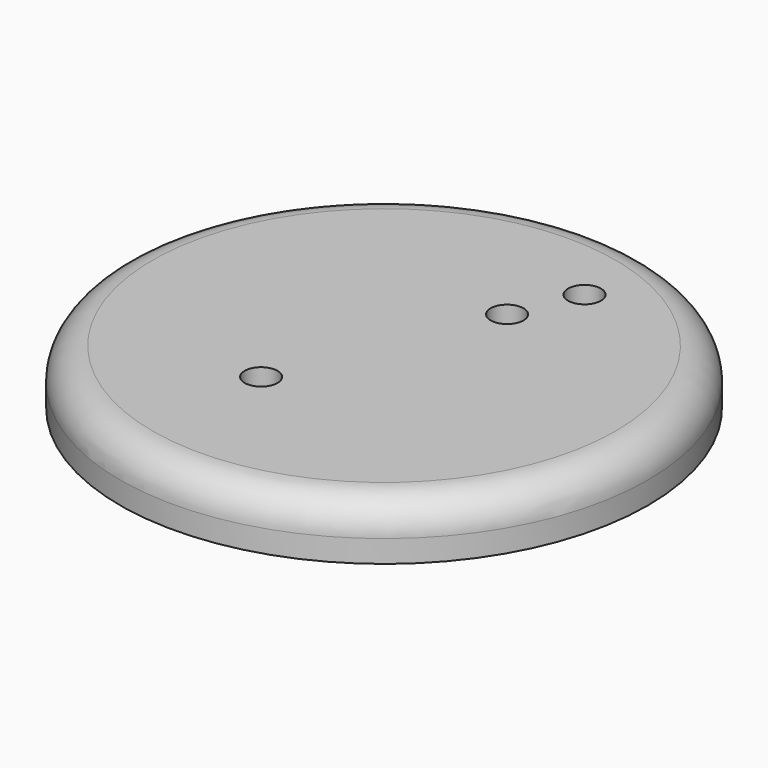
from build123d import *

# Parameters (mm, degrees)
F0_R           = 65
F1_DEPTH       = 15
F2_R           = 8
F3_R           = 60
F3_R_2         = 54
F4_DEPTH       = 3
F5_R           = 8
F6_DEPTH       = 10
F9_R           = 1.5
F10_DEPTH      = 55.0000001083
F10_DEPTH_BACK = 55.0000001083
F11_R          = 1.5
F12_DEPTH      = 55.0000001
F12_DEPTH_BACK = 55.0000000958
F13_R          = 1.5
F14_DEPTH      = 55.0000001083
F14_DEPTH_BACK = 55.0000001083
F15_R          = 1.5
F16_DEPTH      = 55.0000001083
F16_DEPTH_BACK = 55.0000001083
F17_R          = 8
F17_R_2        = 5.75
F18_DEPTH      = 4
F19_R          = 1.75
F20_DEPTH      = 10
F21_R          = 4.05
F22_DEPTH      = 15.001
F23_R          = 8.1
F24_DEPTH      = 7.1
F25_R          = 3.5
F26_DEPTH      = 8
F27_R          = 65
F27_R_2        = 60
F28_DEPTH      = 1.5
F29_SIZE       = 1.49999


# Not quite as in the source:
# - a fillet or chamfer is up to 0.001 mm smaller than in the source, because OpenCascade refuses the exact size


with BuildPart() as f1:
    # F0 (on Top) → F1 (new body)
    with BuildSketch(Plane.XY):
        Circle(F0_R)
    extrude(amount=F1_DEPTH)

    # F2
    f2_edges = [f1.edges().sort_by_distance(p)[0] for p in [
        (-65, 0, 15),
    ]]
    fillet(f2_edges, radius=F2_R)

    # F3 (on face) → F4 (cut)
    with BuildSketch(Plane(origin=(0, 0, 0), x_dir=(1, 0, 0), z_dir=(0, 0, -1))):
        Circle(F3_R)
        Circle(F3_R_2, mode=Mode.SUBTRACT)
    extrude(amount=-F4_DEPTH, mode=Mode.SUBTRACT)

    # F5 (on face) → F6 (cut)
    with BuildSketch(Plane(origin=(0, 0, 0), x_dir=(1, 0, 0), z_dir=(0, 0, -1))):
        Circle(F5_R)
    extrude(amount=-F6_DEPTH, mode=Mode.SUBTRACT)

    # F9 (on Front) → F10 (cut, two sides)
    with BuildSketch(Plane.XZ) as f10_sk:
        Circle(F9_R)
    extrude(amount=-F10_DEPTH, mode=Mode.SUBTRACT)
    extrude(f10_sk.sketch, amount=F10_DEPTH_BACK, mode=Mode.SUBTRACT)

    # F11 (on Right) → F12 (cut, two sides)
    with BuildSketch(Plane.YZ) as f12_sk:
        Circle(F11_R)
    extrude(amount=F12_DEPTH, mode=Mode.SUBTRACT)
    extrude(f12_sk.sketch, amount=-F12_DEPTH_BACK, mode=Mode.SUBTRACT)

    # F13 (on face) → F14 (cut, two sides)
    with BuildSketch(Plane(origin=(0, 0, 0), x_dir=(0.7071067812, -0.7071067812, 0), z_dir=(-0.7071067812, -0.7071067812, 0))) as f14_sk:
        Circle(F13_R)
    extrude(amount=-F14_DEPTH, mode=Mode.SUBTRACT)
    extrude(f14_sk.sketch, amount=F14_DEPTH_BACK, mode=Mode.SUBTRACT)

    # F15 (on face) → F16 (cut, two sides)
    with BuildSketch(Plane(origin=(0, 0, 0), x_dir=(0.7071067812, 0.7071067812, 0), z_dir=(0.7071067812, -0.7071067812, 0))) as f16_sk:
        Circle(F15_R)
    extrude(amount=-F16_DEPTH, mode=Mode.SUBTRACT)
    extrude(f16_sk.sketch, amount=F16_DEPTH_BACK, mode=Mode.SUBTRACT)

    # F17 (on face) → F18 (join)
    with BuildSketch(Plane(origin=(0, 0, 10), x_dir=(1, 0, 0), z_dir=(0, 0, -1))):
        Circle(F17_R)
        Circle(F17_R_2, mode=Mode.SUBTRACT)
    extrude(amount=F18_DEPTH)

    # F19 (on face) → F20 (cut)
    with BuildSketch(Plane(origin=(0, 0, 0), x_dir=(1, 0, 0), z_dir=(0, 0, -1))):
        with Locations((0, 7)):
            Circle(F19_R)
        with Locations((-4.9497474683, 4.9497474683)):
            Circle(F19_R)
        with Locations((-7, 0)):
            Circle(F19_R)
        with Locations((-4.9497474683, -4.9497474683)):
            Circle(F19_R)
        with Locations((0, -7)):
            Circle(F19_R)
        with Locations((4.9497474683, -4.9497474683)):
            Circle(F19_R)
        with Locations((7, 0)):
            Circle(F19_R)
        with Locations((4.9497474683, 4.9497474683)):
            Circle(F19_R)
    extrude(amount=-F20_DEPTH, mode=Mode.SUBTRACT)

    # F21 (on face) → F22 (cut, through all)
    with BuildSketch(Plane(origin=(0, 0, 0), x_dir=(1, 0, 0), z_dir=(0, 0, -1))):
        with Locations((-10.3324526739, 24.9447473778)):
            Circle(F21_R)
        with Locations((10.3324526739, -24.9447473778)):
            Circle(F21_R)
        with Locations((16.8380710241, -40.6506994305)):
            Circle(F21_R)
    extrude(amount=-F22_DEPTH, mode=Mode.SUBTRACT)

    # F23 (on face) → F24 (cut)
    with BuildSketch(Plane(origin=(0, 0, 0), x_dir=(1, 0, 0), z_dir=(0, 0, -1))):
        with Locations((-10.3324526739, 24.9447473778)):
            Circle(F23_R)
        with Locations((10.3324526739, -24.9447473778)):
            Circle(F23_R)
        with Locations((16.8380710241, -40.6506994305)):
            Circle(F23_R)
    extrude(amount=-F24_DEPTH, mode=Mode.SUBTRACT)

    # F25 (on face) → F26 (cut)
    with BuildSketch(Plane(origin=(0, 0, 0), x_dir=(1, 0, 0), z_dir=(0, 0, -1))):
        with Locations((-41.574578963, 17.2207544564)):
            Circle(F25_R)
        with Locations((-17.2207544564, -41.574578963)):
            Circle(F25_R)
        with Locations((41.574578963, -17.2207544564)):
            Circle(F25_R)
        with Locations((17.2207544564, 41.574578963)):
            Circle(F25_R)
    extrude(amount=-F26_DEPTH, mode=Mode.SUBTRACT)

    # F27 (on face) → F28 (cut)
    with BuildSketch(Plane(origin=(0, 0, 0), x_dir=(1, 0, 0), z_dir=(0, 0, -1))):
        Circle(F27_R)
        Circle(F27_R_2, mode=Mode.SUBTRACT)
    extrude(amount=-F28_DEPTH, mode=Mode.SUBTRACT)

    # F29 (size 1.5 in the source; OpenCascade refuses exactly that, so slightly less here)
    f29_edges = [f1.edges().sort_by_distance(p)[0] for p in [
        (-49.889495, -20.664905, 0),
        (49.889495, -20.664905, 0),
        (20.664905, -49.889495, 0),
        (-20.664905, -49.889495, 0),
        (-49.889495, 20.664905, 0),
        (-20.664905, 49.889495, 0),
        (20.664905, 49.889495, 0),
        (49.889495, 20.664905, 0),
    ]]
    chamfer(f29_edges, length=F29_SIZE)


solid = f1.part
